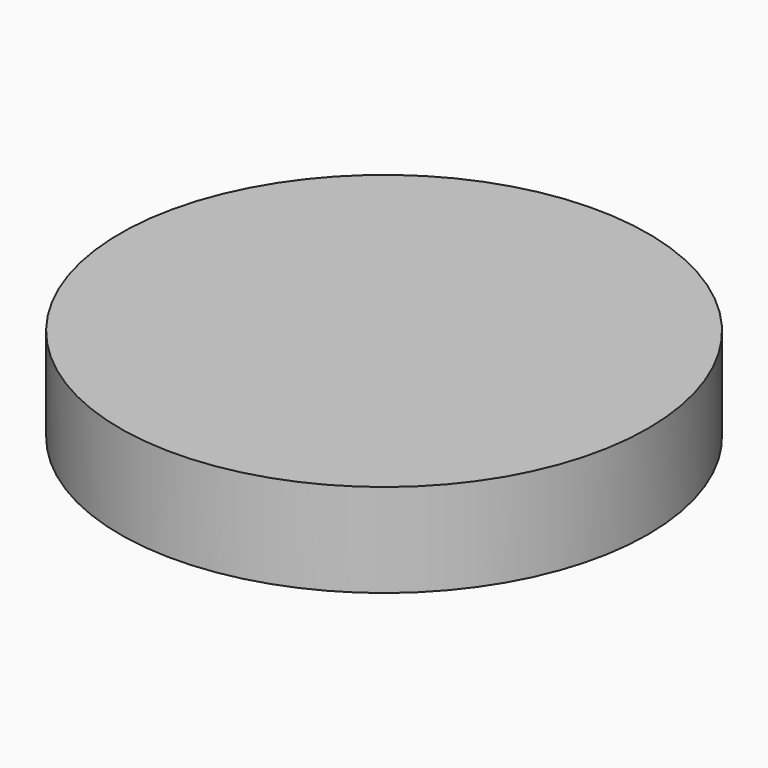
from build123d import *

# Parameters (mm, degrees)
F2_R     = 71.8376389327
F3_DEPTH = 25.4


# Not quite as in the source:
# - the program builds the solid bodies; features that only make, move or delete a surface that nothing else refers to are left out


with BuildPart() as f3:
    # F2 (on Top) → F3 (new body)
    with BuildSketch(Plane.XY):
        Circle(F2_R)
    extrude(amount=F3_DEPTH)


solid = f3.part
